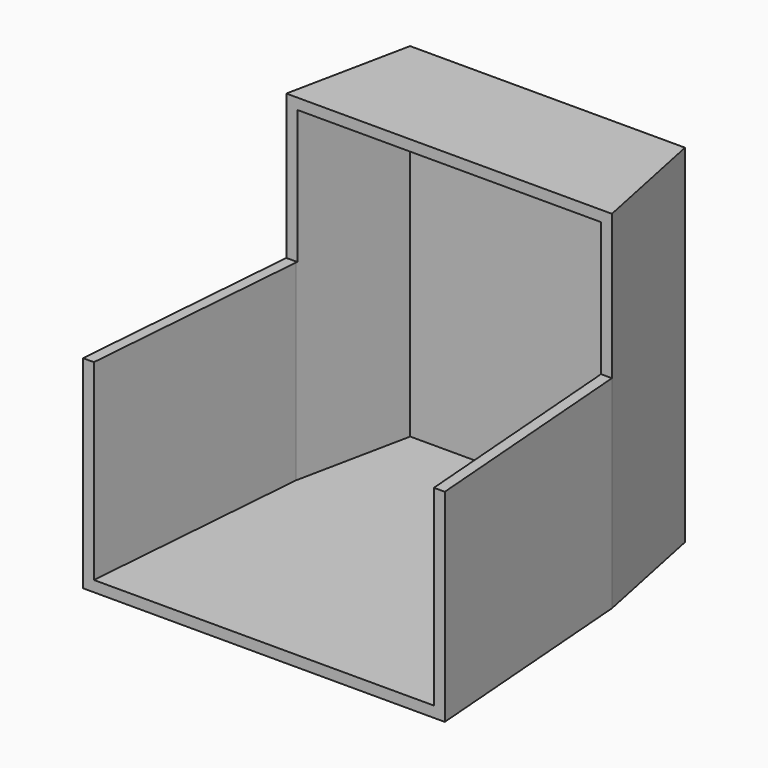
from build123d import *

# Parameters (mm, degrees)
F1_DEPTH = 48
F3_DEPTH = 20
F4_T     = 1.5


# Not quite as in the source:
# - a shell that OpenCascade refuses in one call is made with other operations: the cavity is built on its own and cut out


with BuildPart() as f1:
    # F0 (on Top) → F1 (new body)
    with BuildSketch(Plane.XY):
        Polygon((22.5, 22.8382229426), (-22.5, 22.8382229426), (-25, -9.1617770574), (25, -9.1617770574), align=None)
        Polygon((19, 39.8382229426), (-19, 39.8382229426), (-22.5, 22.8382229426), (22.5, 22.8382229426), align=None)
    extrude(amount=F1_DEPTH)

    # F2 (on face) → F3 (cut)
    with BuildSketch(Plane.XY.offset(48)):
        Polygon((22.5, 22.8382229426), (-22.5, 22.8382229426), (-25, -9.1617770574), (25, -9.1617770574), align=None)
    extrude(amount=-F3_DEPTH, mode=Mode.SUBTRACT)

    # F4: shell of thickness 1.5, made by hand


with BuildPart() as f4_core1:
    # F4_t2: copy of F1
    add(f1.part)

    # the walls: a layer under each face that stays
    f4_faces = [f4_core1.faces().sort_by_distance(p)[0] for p in [
        (0, 15.3382229426, 0),
        (23.75, 6.8382229426, 14),
        (-23.75, 6.8382229426, 14),
        (20.75, 31.3382229426, 24),
        (0, 39.8382229426, 24),
        (-20.75, 31.3382229426, 24),
        (0, 31.3382229426, 48),
    ]]
    thicken(f4_faces, amount=-F4_T, mode=Mode.SUBTRACT)


with BuildPart() as f1_1:
    add(f1.part)

    # what is left inside the walls is the cavity
    f4_cavity = [f4_core1.part.solids().sort_by_distance(p)[0] for p in [
        (0, 6.671556, 1.515),
    ]]
    add(f4_cavity, mode=Mode.SUBTRACT)


solid = f1_1.part
